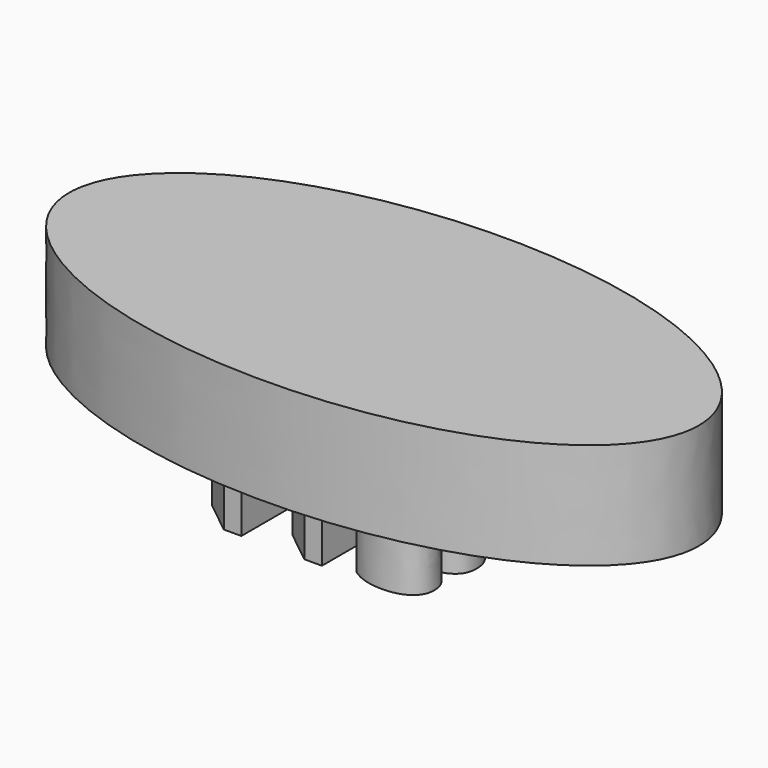
from build123d import *

# Parameters (mm, degrees)
F1_DEPTH     = 25.4
F2_TEXT_SIZE = 33.7983882572
F3_DEPTH     = 25.4


# Not quite as in the source:
# - Text() gives the source's letters only with a copy of the font that has no kerning and outlines rounded to 1/6400 em; it was checked with that copy


with BuildPart() as f1:
    # F0 (on Top) → F1 (new body)
    with BuildSketch(Plane.XY):
        with BuildLine():
            add(Edge.make_bspline(
                [(-75.4115581512, 0), (-75.4115581512, -63.5307320408), (37.7057790756, -31.7653660204), (150.8231163025, 0), (37.7057790756, 31.7653660204), (-75.4115581512, 63.5307320408), (-75.4115581512, 0)],
                knots=[0, 0, 0, 2.0943951024, 2.0943951024, 4.1887902048, 4.1887902048, 6.2831853072, 6.2831853072, 6.2831853072], degree=2, weights=[1, 0.5, 1, 0.5, 1, 0.5, 1]))
        make_face()
    extrude(amount=F1_DEPTH)

    # F2 (on face) → F3 (join)
    with BuildSketch(Plane(origin=(0, 0, 0), x_dir=(1, 0, 0), z_dir=(0, 0, -1))):
        with Locations((-38.3462645113, -11.9146313518)):
            Text('113', F2_TEXT_SIZE, font='Open Sans', font_style=FontStyle.BOLD, text_align=(TextAlign.LEFT, TextAlign.BOTTOM))
    extrude(amount=F3_DEPTH)


solid = f1.part
